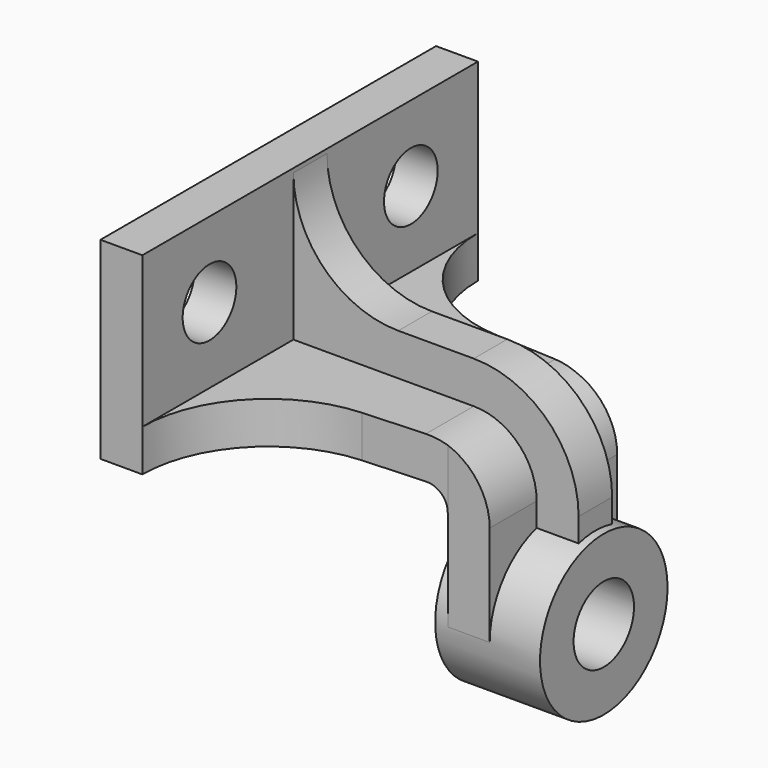
from build123d import *

# Parameters (mm, degrees)
F1_DEPTH    = 50
F2_DEPTH    = 19
F4_DEPTH    = 10
F5_R        = 5
F6_T1_DEPTH = 113
F7_R        = 8
F8_DEPTH    = 10
F11_W       = 28.4062897359
F11_H       = 10.0000000002
F12_DEPTH   = 5
F10_R       = 9
F13_DEPTH   = 25
F14_DEPTH   = 20


# Not quite as in the source:
# - a fillet or chamfer that OpenCascade refuses, or shapes differently, is made with other operations: its cross-section is extruded or revolved along the edge and cut away or added


with BuildPart() as f1:
    # F0 (on Front) → F1 (new body, symmetric)
    with BuildSketch(Plane.XZ):
        Polygon((0, 46), (0, 0), (58, 0), (58, 10), (10, 10), (10, 46), align=None)
    extrude(amount=F1_DEPTH, both=True)

    # F0 (on Front) → F2 (join, symmetric)
    with BuildSketch(Plane.XZ):
        Polygon((0, 46), (0, 0), (58, 0), (58, 10), (10, 10), (10, 46), align=None)
        Polygon((58, 10), (58, 0), (58, -29), (68, -29), (68, 10), align=None)
    extrude(amount=F2_DEPTH, both=True)

    # F3 (on face) → F4 (cut, through all)
    with BuildSketch(Plane.XY.offset(10)):
        with BuildLine():
            Line((58, -19), (38.4062897359, -20.0423617821))
            ThreePointArc((38.4062897359, -20.0423617821), (18.2306257793, -29.3579471457), (10, -50))
            Line((10, -50), (58, -50))
            Line((58, -50), (58, -19))
        make_face()
        with BuildLine():
            Line((58, 50), (10, 50))
            ThreePointArc((10, 50), (18.2306257793, 29.3579471457), (38.4062897359, 20.0423617821))
            Line((38.4062897359, 20.0423617821), (58, 19))
            Line((58, 19), (58, 50))
        make_face()
    extrude(amount=-F4_DEPTH, mode=Mode.SUBTRACT)

    # F5
    f5_edges = [f1.edges().sort_by_distance(p)[0] for p in [
        (58, 0, 0),
    ]]
    fillet(f5_edges, radius=F5_R)

    # F6: fillet of radius 15 on 1 edges, made by hand

    # F6_s2 → F6_t1 (cut)
    with BuildSketch(Plane.XZ.offset(-56.5)):
        with BuildLine():
            ThreePointArc((53, 10), (63.6066017178, 5.6066017178), (68, -5))
            Line((68, -5), (68, 10))
            Line((68, 10), (53, 10))
        make_face()
    extrude(amount=F6_T1_DEPTH, mode=Mode.SUBTRACT)

    # F7 (on face) → F8 (cut, through all)
    with BuildSketch(Plane.YZ.offset(10)):
        with Locations((-30, 28)):
            Circle(F7_R)
        with Locations((30, 28)):
            Circle(F7_R)
    extrude(amount=-F8_DEPTH, mode=Mode.SUBTRACT)

    # F11 (on Front) → F12 (join, symmetric)
    with BuildSketch(Plane.XZ):
        Polygon((10, 10), (10, 45.0000000683), (10, 46), (0, 46), (0, 0), (10, 0), align=None)
        with BuildLine():
            ThreePointArc((35, 20), (17.3223304462, 27.3223304945), (10, 45.0000000683))
            Line((10, 45.0000000683), (10, 10))
            Line((10, 10), (38.4062897359, 10))
            Line((38.4062897359, 10), (53, 10))
            ThreePointArc((53, 10), (55.5365296809, 9.7839783948), (58, 9.1421356237))
            ThreePointArc((58, 9.1421356237), (65.2474487139, 3.6602540378), (68, -5))
            Line((68, -5), (68, -29))
            Line((68, -29), (78, -29))
            Line((78, -29), (78, -5))
            ThreePointArc((78, -5), (70.6776695297, 12.6776695297), (53, 20))
            Line((53, 20), (35, 20))
        make_face()
        with Locations((24.2031448679, 4.9999999999)):
            Rectangle(F11_W, F11_H)
    extrude(amount=F12_DEPTH, both=True)

    # F10 (on offset) → F13 (join)
    with BuildSketch(Plane.YZ.offset(80)):
        with BuildLine():
            ThreePointArc((-19, -29), (0, -48), (19, -29))
            ThreePointArc((19, -29), (0, -10), (-19, -29))
        make_face()
        with Locations((0, -29)):
            Circle(F10_R, mode=Mode.SUBTRACT)
    extrude(amount=-F13_DEPTH)

    # F14 (cut, through all): faces of the model
    f14_faces = [f1.faces().sort_by_distance(p)[0] for p in [
        (78, 0, -24.7319215604),
        (68, -6.6350234662, -26.0867467093),
        (68, 6.6350234662, -26.0867467093),
    ]]
    extrude(f14_faces, amount=-F14_DEPTH, mode=Mode.SUBTRACT)


solid = f1.part
